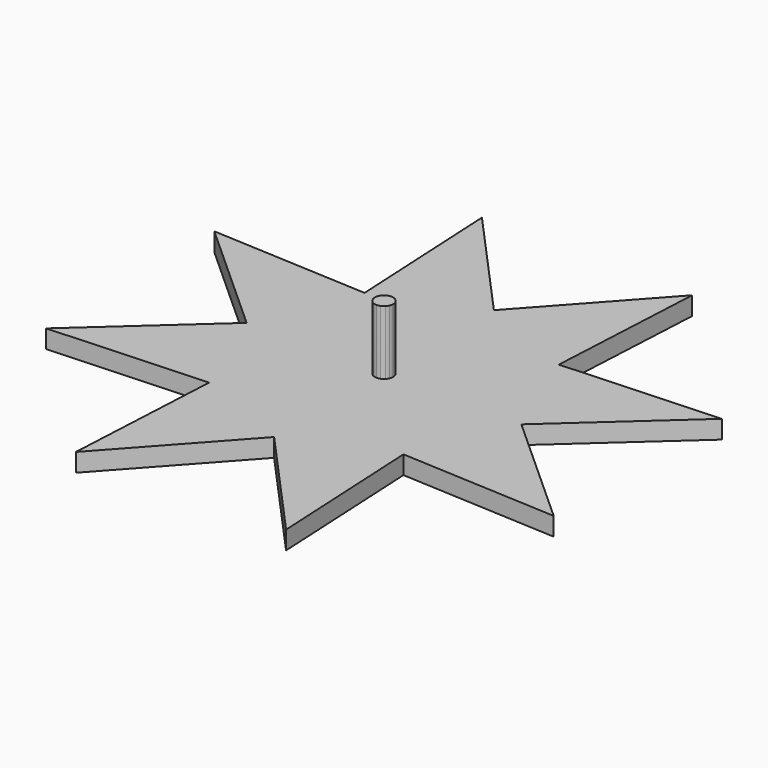
from build123d import *

# Parameters (mm, degrees)
F1_DEPTH = 5.08
F2_DEPTH = 22.86


# Not quite as in the source:
# - a feature names something its author has since deleted; it is built from what else it names


with BuildPart() as f1:
    # F0 (on Top) → F1 (new body)
    with BuildSketch(Plane.XY):
        with BuildLine():
            Line((-70.3996203774, -29.1604775462), (-26.9407683632, -26.9407683632))
            ThreePointArc((-26.9407683632, -26.9407683632), (-31.6789922287, -21.167225878), (-35.1998101887, -14.5802387731))
            Line((-35.1998101887, -14.5802387731), (-70.3996203774, -29.1604775462))
        make_face()
        with BuildLine():
            ThreePointArc((-35.1998101887, -14.5802387731), (-37.3679191834, -7.4329412688), (-38.1, 0))
            Line((-38.1, 0), (-70.3996203774, -29.1604775462))
            Line((-70.3996203774, -29.1604775462), (-35.1998101887, -14.5802387731))
        make_face()
        with BuildLine():
            Line((-70.3996203774, 29.1604775462), (-38.1, 0))
            ThreePointArc((-38.1, 0), (-37.3679191834, 7.4329412688), (-35.1998101887, 14.5802387731))
            Line((-35.1998101887, 14.5802387731), (-70.3996203774, 29.1604775462))
        make_face()
        with BuildLine():
            ThreePointArc((-35.1998101887, 14.5802387731), (-31.6789922287, 21.167225878), (-26.9407683632, 26.9407683632))
            Line((-26.9407683632, 26.9407683632), (-70.3996203774, 29.1604775462))
            Line((-70.3996203774, 29.1604775462), (-35.1998101887, 14.5802387731))
        make_face()
        with BuildLine():
            Line((-14.5802387731, 35.1998101887), (-29.1604775462, 70.3996203774))
            Line((-29.1604775462, 70.3996203774), (-26.9407683632, 26.9407683632))
            ThreePointArc((-26.9407683632, 26.9407683632), (-21.167225878, 31.6789922287), (-14.5802387731, 35.1998101887))
        make_face()
        with BuildLine():
            ThreePointArc((-14.5802387731, 35.1998101887), (-7.4329412688, 37.3679191834), (0, 38.1))
            Line((0, 38.1), (-29.1604775462, 70.3996203774))
            Line((-29.1604775462, 70.3996203774), (-14.5802387731, 35.1998101887))
        make_face()
        with BuildLine():
            Line((14.5802387731, 35.1998101887), (29.1604775462, 70.3996203774))
            Line((29.1604775462, 70.3996203774), (0, 38.1))
            ThreePointArc((0, 38.1), (7.4329412688, 37.3679191834), (14.5802387731, 35.1998101887))
        make_face()
        with BuildLine():
            ThreePointArc((14.5802387731, 35.1998101887), (21.167225878, 31.6789922287), (26.9407683632, 26.9407683632))
            Line((26.9407683632, 26.9407683632), (29.1604775462, 70.3996203774))
            Line((29.1604775462, 70.3996203774), (14.5802387731, 35.1998101887))
        make_face()
        with BuildLine():
            Line((38.1, 0), (70.3996203774, 29.1604775462))
            Line((70.3996203774, 29.1604775462), (35.1998101887, 14.5802387731))
            ThreePointArc((35.1998101887, 14.5802387731), (37.3679191834, 7.4329412688), (38.1, 0))
        make_face()
        with BuildLine():
            Line((35.1998101887, -14.5802387731), (70.3996203774, -29.1604775462))
            Line((70.3996203774, -29.1604775462), (38.1, 0))
            ThreePointArc((38.1, 0), (37.3679191834, -7.4329412688), (35.1998101887, -14.5802387731))
        make_face()
        with BuildLine():
            Line((26.9407683632, -26.9407683632), (70.3996203774, -29.1604775462))
            Line((70.3996203774, -29.1604775462), (35.1998101887, -14.5802387731))
            ThreePointArc((35.1998101887, -14.5802387731), (31.6789922287, -21.167225878), (26.9407683632, -26.9407683632))
        make_face()
        with BuildLine():
            Line((29.1604775462, -70.3996203774), (26.9407683632, -26.9407683632))
            ThreePointArc((26.9407683632, -26.9407683632), (21.167225878, -31.6789922287), (14.5802387731, -35.1998101887))
            Line((14.5802387731, -35.1998101887), (29.1604775462, -70.3996203774))
        make_face()
        with BuildLine():
            Line((0, -38.1), (29.1604775462, -70.3996203774))
            Line((29.1604775462, -70.3996203774), (14.5802387731, -35.1998101887))
            ThreePointArc((14.5802387731, -35.1998101887), (7.4329412688, -37.3679191834), (0, -38.1))
        make_face()
        with BuildLine():
            Line((-29.1604775462, -70.3996203774), (0, -38.1))
            ThreePointArc((0, -38.1), (-7.4329412688, -37.3679191834), (-14.5802387731, -35.1998101887))
            Line((-14.5802387731, -35.1998101887), (-29.1604775462, -70.3996203774))
        make_face()
        with BuildLine():
            Line((-26.9407683632, -26.9407683632), (-29.1604775462, -70.3996203774))
            Line((-29.1604775462, -70.3996203774), (-14.5802387731, -35.1998101887))
            ThreePointArc((-14.5802387731, -35.1998101887), (-21.167225878, -31.6789922287), (-26.9407683632, -26.9407683632))
        make_face()
        with BuildLine():
            ThreePointArc((-0.9720159182, -2.3466540126), (-1.4111483919, -2.1119328152), (-1.7960512242, -1.7960512242))
            Line((-1.7960512242, -1.7960512242), (-26.9407683632, -26.9407683632))
            ThreePointArc((-26.9407683632, -26.9407683632), (-21.167225878, -31.6789922287), (-14.5802387731, -35.1998101887))
            Line((-14.5802387731, -35.1998101887), (-0.9720159182, -2.3466540126))
        make_face()
        with BuildLine():
            ThreePointArc((-14.5802387731, -35.1998101887), (-7.4329412688, -37.3679191834), (0, -38.1))
            Line((0, -38.1), (0, -2.54))
            ThreePointArc((0, -2.54), (-0.4955294179, -2.4911946122), (-0.9720159182, -2.3466540126))
            Line((-0.9720159182, -2.3466540126), (-14.5802387731, -35.1998101887))
        make_face()
        with BuildLine():
            ThreePointArc((0, -38.1), (7.4329412688, -37.3679191834), (14.5802387731, -35.1998101887))
            Line((14.5802387731, -35.1998101887), (0.9720159182, -2.3466540126))
            ThreePointArc((0.9720159182, -2.3466540126), (0.4955294179, -2.4911946122), (0, -2.54))
            Line((0, -2.54), (0, -38.1))
        make_face()
        with BuildLine():
            ThreePointArc((14.5802387731, -35.1998101887), (21.167225878, -31.6789922287), (26.9407683632, -26.9407683632))
            Line((26.9407683632, -26.9407683632), (1.7960512242, -1.7960512242))
            ThreePointArc((1.7960512242, -1.7960512242), (1.4111483919, -2.1119328152), (0.9720159182, -2.3466540126))
            Line((0.9720159182, -2.3466540126), (14.5802387731, -35.1998101887))
        make_face()
        with BuildLine():
            ThreePointArc((26.9407683632, -26.9407683632), (31.6789922287, -21.167225878), (35.1998101887, -14.5802387731))
            Line((35.1998101887, -14.5802387731), (2.3466540126, -0.9720159182))
            ThreePointArc((2.3466540126, -0.9720159182), (2.1119328152, -1.4111483919), (1.7960512242, -1.7960512242))
            Line((1.7960512242, -1.7960512242), (26.9407683632, -26.9407683632))
        make_face()
        with BuildLine():
            ThreePointArc((35.1998101887, -14.5802387731), (37.3679191834, -7.4329412688), (38.1, 0))
            Line((38.1, 0), (2.54, 0))
            ThreePointArc((2.54, 0), (2.4911946122, -0.4955294179), (2.3466540126, -0.9720159182))
            Line((2.3466540126, -0.9720159182), (35.1998101887, -14.5802387731))
        make_face()
        with BuildLine():
            Line((2.54, 0), (38.1, 0))
            ThreePointArc((38.1, 0), (37.3679191834, 7.4329412688), (35.1998101887, 14.5802387731))
            Line((35.1998101887, 14.5802387731), (2.3466540126, 0.9720159182))
            ThreePointArc((2.3466540126, 0.9720159182), (2.4911946122, 0.4955294179), (2.54, 0))
        make_face()
        with BuildLine():
            Line((2.3466540126, 0.9720159182), (35.1998101887, 14.5802387731))
            ThreePointArc((35.1998101887, 14.5802387731), (31.6789922287, 21.167225878), (26.9407683632, 26.9407683632))
            Line((26.9407683632, 26.9407683632), (1.7960512242, 1.7960512242))
            ThreePointArc((1.7960512242, 1.7960512242), (2.1119328152, 1.4111483919), (2.3466540126, 0.9720159182))
        make_face()
        with BuildLine():
            Line((1.7960512242, 1.7960512242), (26.9407683632, 26.9407683632))
            ThreePointArc((26.9407683632, 26.9407683632), (21.167225878, 31.6789922287), (14.5802387731, 35.1998101887))
            Line((14.5802387731, 35.1998101887), (0.9720159182, 2.3466540126))
            ThreePointArc((0.9720159182, 2.3466540126), (1.4111483919, 2.1119328152), (1.7960512242, 1.7960512242))
        make_face()
        with BuildLine():
            Line((0.9720159182, 2.3466540126), (14.5802387731, 35.1998101887))
            ThreePointArc((14.5802387731, 35.1998101887), (7.4329412688, 37.3679191834), (0, 38.1))
            Line((0, 38.1), (0, 2.54))
            ThreePointArc((0, 2.54), (0.4955294179, 2.4911946122), (0.9720159182, 2.3466540126))
        make_face()
        with BuildLine():
            Line((0, 2.54), (0, 38.1))
            ThreePointArc((0, 38.1), (-7.4329412688, 37.3679191834), (-14.5802387731, 35.1998101887))
            Line((-14.5802387731, 35.1998101887), (-0.9720159182, 2.3466540126))
            ThreePointArc((-0.9720159182, 2.3466540126), (-0.4955294179, 2.4911946122), (0, 2.54))
        make_face()
        with BuildLine():
            Line((-26.9407683632, 26.9407683632), (-1.7960512242, 1.7960512242))
            ThreePointArc((-1.7960512242, 1.7960512242), (-1.4111483919, 2.1119328152), (-0.9720159182, 2.3466540126))
            Line((-0.9720159182, 2.3466540126), (-14.5802387731, 35.1998101887))
            ThreePointArc((-14.5802387731, 35.1998101887), (-21.167225878, 31.6789922287), (-26.9407683632, 26.9407683632))
        make_face()
        with BuildLine():
            ThreePointArc((-2.3466540126, 0.9720159182), (-2.1119328152, 1.4111483919), (-1.7960512242, 1.7960512242))
            Line((-1.7960512242, 1.7960512242), (-26.9407683632, 26.9407683632))
            ThreePointArc((-26.9407683632, 26.9407683632), (-31.6789922287, 21.167225878), (-35.1998101887, 14.5802387731))
            Line((-35.1998101887, 14.5802387731), (-2.3466540126, 0.9720159182))
        make_face()
        with BuildLine():
            Line((-38.1, 0), (-2.54, 0))
            ThreePointArc((-2.54, 0), (-2.4911946122, 0.4955294179), (-2.3466540126, 0.9720159182))
            Line((-2.3466540126, 0.9720159182), (-35.1998101887, 14.5802387731))
            ThreePointArc((-35.1998101887, 14.5802387731), (-37.3679191834, 7.4329412688), (-38.1, 0))
        make_face()
        with BuildLine():
            ThreePointArc((-2.3466540126, -0.9720159182), (-2.4911946122, -0.4955294179), (-2.54, 0))
            Line((-2.54, 0), (-38.1, 0))
            ThreePointArc((-38.1, 0), (-37.3679191834, -7.4329412688), (-35.1998101887, -14.5802387731))
            Line((-35.1998101887, -14.5802387731), (-2.3466540126, -0.9720159182))
        make_face()
        with BuildLine():
            Line((-26.9407683632, -26.9407683632), (-1.7960512242, -1.7960512242))
            ThreePointArc((-1.7960512242, -1.7960512242), (-2.1119328152, -1.4111483919), (-2.3466540126, -0.9720159182))
            Line((-2.3466540126, -0.9720159182), (-35.1998101887, -14.5802387731))
            ThreePointArc((-35.1998101887, -14.5802387731), (-31.6789922287, -21.167225878), (-26.9407683632, -26.9407683632))
        make_face()
        with BuildLine():
            Line((35.1998101887, 14.5802387731), (70.3996203774, 29.1604775462))
            Line((70.3996203774, 29.1604775462), (26.9407683632, 26.9407683632))
            ThreePointArc((26.9407683632, 26.9407683632), (31.6789922287, 21.167225878), (35.1998101887, 14.5802387731))
        make_face()
    extrude(amount=F1_DEPTH)

    # F0 (on Top) → F2 (join)
    with BuildSketch(Plane.XY):
        with BuildLine():
            Line((-1.7960512242, 1.7960512242), (0, 0))
            Line((0, 0), (-0.9720159182, 2.3466540126))
            ThreePointArc((-0.9720159182, 2.3466540126), (-1.4111483919, 2.1119328152), (-1.7960512242, 1.7960512242))
        make_face()
        with BuildLine():
            Line((-2.3466540126, 0.9720159182), (0, 0))
            Line((0, 0), (-1.7960512242, 1.7960512242))
            ThreePointArc((-1.7960512242, 1.7960512242), (-2.1119328152, 1.4111483919), (-2.3466540126, 0.9720159182))
        make_face()
        with BuildLine():
            Line((-2.54, 0), (0, 0))
            Line((0, 0), (-2.3466540126, 0.9720159182))
            ThreePointArc((-2.3466540126, 0.9720159182), (-2.4911946122, 0.4955294179), (-2.54, 0))
        make_face()
        with BuildLine():
            Line((-2.3466540126, -0.9720159182), (0, 0))
            Line((0, 0), (-2.54, 0))
            ThreePointArc((-2.54, 0), (-2.4911946122, -0.4955294179), (-2.3466540126, -0.9720159182))
        make_face()
        with BuildLine():
            Line((-1.7960512242, -1.7960512242), (0, 0))
            Line((0, 0), (-2.3466540126, -0.9720159182))
            ThreePointArc((-2.3466540126, -0.9720159182), (-2.1119328152, -1.4111483919), (-1.7960512242, -1.7960512242))
        make_face()
        with BuildLine():
            Line((-0.9720159182, -2.3466540126), (0, 0))
            Line((0, 0), (-1.7960512242, -1.7960512242))
            ThreePointArc((-1.7960512242, -1.7960512242), (-1.4111483919, -2.1119328152), (-0.9720159182, -2.3466540126))
        make_face()
        with BuildLine():
            Line((0, -2.54), (0, 0))
            Line((0, 0), (-0.9720159182, -2.3466540126))
            ThreePointArc((-0.9720159182, -2.3466540126), (-0.4955294179, -2.4911946122), (0, -2.54))
        make_face()
        with BuildLine():
            Line((0.9720159182, -2.3466540126), (0, 0))
            Line((0, 0), (0, -2.54))
            ThreePointArc((0, -2.54), (0.4955294179, -2.4911946122), (0.9720159182, -2.3466540126))
        make_face()
        with BuildLine():
            ThreePointArc((0.9720159182, -2.3466540126), (1.4111483919, -2.1119328152), (1.7960512242, -1.7960512242))
            Line((1.7960512242, -1.7960512242), (0, 0))
            Line((0, 0), (0.9720159182, -2.3466540126))
        make_face()
        with BuildLine():
            ThreePointArc((1.7960512242, -1.7960512242), (2.1119328152, -1.4111483919), (2.3466540126, -0.9720159182))
            Line((2.3466540126, -0.9720159182), (0, 0))
            Line((0, 0), (1.7960512242, -1.7960512242))
        make_face()
        with BuildLine():
            ThreePointArc((2.3466540126, -0.9720159182), (2.4911946122, -0.4955294179), (2.54, 0))
            Line((2.54, 0), (0, 0))
            Line((0, 0), (2.3466540126, -0.9720159182))
        make_face()
        with BuildLine():
            Line((0, 0), (2.54, 0))
            ThreePointArc((2.54, 0), (2.4911946122, 0.4955294179), (2.3466540126, 0.9720159182))
            Line((2.3466540126, 0.9720159182), (0, 0))
        make_face()
        with BuildLine():
            Line((0, 0), (2.3466540126, 0.9720159182))
            ThreePointArc((2.3466540126, 0.9720159182), (2.1119328152, 1.4111483919), (1.7960512242, 1.7960512242))
            Line((1.7960512242, 1.7960512242), (0, 0))
        make_face()
        with BuildLine():
            Line((0, 2.54), (0, 0))
            Line((0, 0), (0.9720159182, 2.3466540126))
            ThreePointArc((0.9720159182, 2.3466540126), (0.4955294179, 2.4911946122), (0, 2.54))
        make_face()
        with BuildLine():
            Line((-0.9720159182, 2.3466540126), (0, 0))
            Line((0, 0), (0, 2.54))
            ThreePointArc((0, 2.54), (-0.4955294179, 2.4911946122), (-0.9720159182, 2.3466540126))
        make_face()
        with BuildLine():
            Line((0, 0), (1.7960512242, 1.7960512242))
            ThreePointArc((1.7960512242, 1.7960512242), (1.4111483919, 2.1119328152), (0.9720159182, 2.3466540126))
            Line((0.9720159182, 2.3466540126), (0, 0))
        make_face()
    extrude(amount=F2_DEPTH)


solid = f1.part
